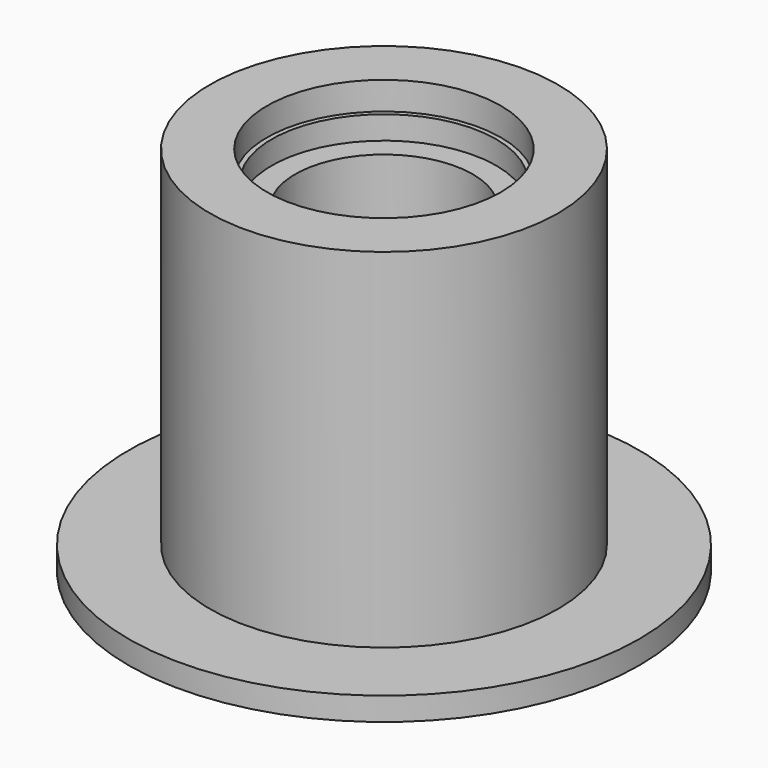
from build123d import *

# Parameters (mm, degrees)
F0_R         = 11
F1_DEPTH     = 1
F2_R         = 7.5
F3_DEPTH     = 15
F4_R         = 3.825
F5_DEPTH     = 25
F6_R         = 5.95
F7_DEPTH     = 7.3
F8_R         = 5.0375
F8_R_2       = 3.825
F9_DEPTH     = 1.2
F10_S5_R     = 5.95
F10_T6_DEPTH = 10
F11_R        = 4.834999796
F11_R_2      = 3.825
F12_DEPTH    = 1


# Not quite as in the source:
# - a fillet or chamfer that OpenCascade refuses, or shapes differently, is made with other operations: its cross-section is extruded or revolved along the edge and cut away or added


with BuildPart() as f1:
    # F0 (on Top) → F1 (new body)
    with BuildSketch(Plane.XY):
        Circle(F0_R)
    extrude(amount=F1_DEPTH)

    # F2 (on face) → F3 (join)
    with BuildSketch(Plane.XY.offset(1)):
        Circle(F2_R)
    extrude(amount=F3_DEPTH)

    # F4 (on face) → F5 (cut)
    with BuildSketch(Plane.XY.offset(16)):
        Circle(F4_R)
    extrude(amount=-F5_DEPTH, mode=Mode.SUBTRACT)

    # F6 (on face) → F7 (cut)
    with BuildSketch(Plane(origin=(0, 0, 0), x_dir=(1, 0, 0), z_dir=(0, 0, -1))):
        Circle(F6_R)
    extrude(amount=-F7_DEPTH, mode=Mode.SUBTRACT)

    # F8 (on face) → F9 (cut)
    with BuildSketch(Plane.XY.offset(16)):
        Circle(F8_R)
        Circle(F8_R_2, mode=Mode.SUBTRACT)
    extrude(amount=-F9_DEPTH, mode=Mode.SUBTRACT)

    # F10: chamfer of 2.2 x 2 on 1 edges, made by hand


with BuildPart() as f10_tool2:
    # F10_s3 → F10_t4 (revolve)
    with BuildSketch(Plane.XZ):
        Polygon((6.025, 7.3), (3.825, 9.3), (3.825, 7.3), align=None)
    revolve(axis=Axis((0, 0, 7.3), (0, 0, 1)))

    # F10_s5 → F10_t6 (intersect, symmetric)
    with BuildSketch(Plane.XY.offset(8.3)):
        Circle(F10_S5_R)
    extrude(amount=F10_T6_DEPTH, both=True, mode=Mode.INTERSECT)


with BuildPart() as f1_1:
    add(f1.part)

    # F10_t1: cut F10_tool2
    add(f10_tool2.part, mode=Mode.SUBTRACT)

    # F11 (on face) → F12 (cut)
    with BuildSketch(Plane.XY.offset(14.8)):
        Circle(F11_R)
        Circle(F11_R_2, mode=Mode.SUBTRACT)
    extrude(amount=-F12_DEPTH, mode=Mode.SUBTRACT)


solid = f1_1.part
